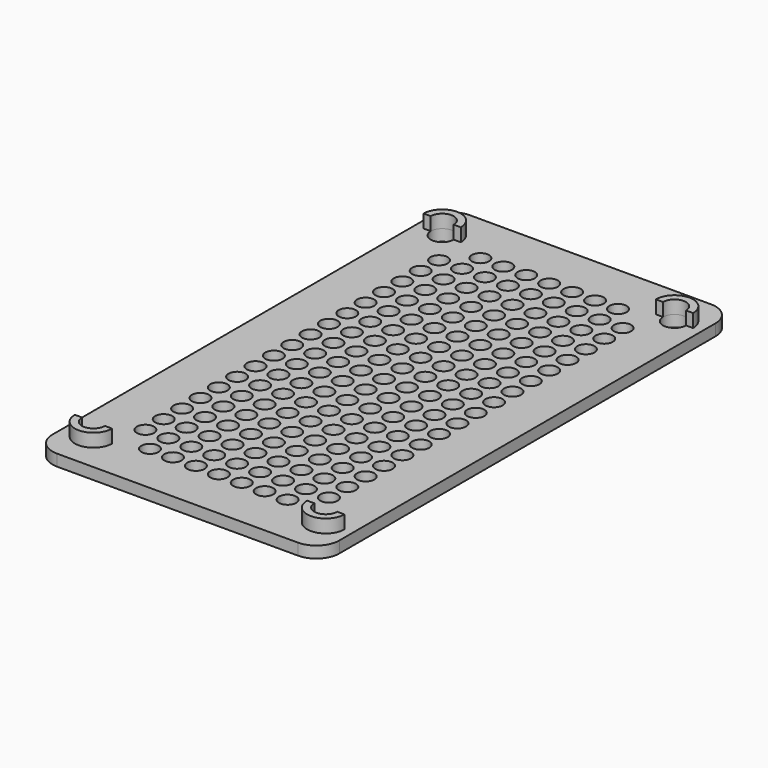
from build123d import *
from build123d import SkipClean  # not in build123d's __all__

# Parameters (mm, degrees)
F0_R     = 2
F0_R_2   = 1.5
F1_DEPTH = 2
F3_DEPTH = 2.3


with BuildPart() as f1:
    # F0 (on Top) → F1 (new body)
    with BuildSketch(Plane.XY):
        with BuildLine():
            Line((-21, -45), (21, -45))
            ThreePointArc((21, -45), (23.8284271247, -43.8284271247), (25, -41))
            Line((25, -41), (25, 41))
            ThreePointArc((25, 41), (23.8284271247, 43.8284271247), (21, 45))
            Line((21, 45), (-21, 45))
            ThreePointArc((-21, 45), (-23.8284271247, 43.8284271247), (-25, 41))
            Line((-25, 41), (-25, -41))
            ThreePointArc((-25, -41), (-23.8284271247, -43.8284271247), (-21, -45))
        make_face()
        with Locations((-20.25, -38)):
            Circle(F0_R, mode=Mode.SUBTRACT)
        with Locations((-16, -32)):
            Circle(F0_R_2, mode=Mode.SUBTRACT)
        with Locations((-16, -28)):
            Circle(F0_R_2, mode=Mode.SUBTRACT)
        with Locations((-16, -24)):
            Circle(F0_R_2, mode=Mode.SUBTRACT)
        with Locations((-12, -36)):
            Circle(F0_R_2, mode=Mode.SUBTRACT)
        with Locations((-8, -36)):
            Circle(F0_R_2, mode=Mode.SUBTRACT)
        with Locations((-4, -36)):
            Circle(F0_R_2, mode=Mode.SUBTRACT)
        with Locations((-12, -32)):
            Circle(F0_R_2, mode=Mode.SUBTRACT)
        with Locations((-8, -32)):
            Circle(F0_R_2, mode=Mode.SUBTRACT)
        with Locations((-12, -28)):
            Circle(F0_R_2, mode=Mode.SUBTRACT)
        with Locations((-12, -24)):
            Circle(F0_R_2, mode=Mode.SUBTRACT)
        with Locations((-8, -28)):
            Circle(F0_R_2, mode=Mode.SUBTRACT)
        with Locations((-8, -24)):
            Circle(F0_R_2, mode=Mode.SUBTRACT)
        with Locations((-4, -32)):
            Circle(F0_R_2, mode=Mode.SUBTRACT)
        with Locations((-4, -28)):
            Circle(F0_R_2, mode=Mode.SUBTRACT)
        with Locations((-4, -24)):
            Circle(F0_R_2, mode=Mode.SUBTRACT)
        with Locations((-16, -20)):
            Circle(F0_R_2, mode=Mode.SUBTRACT)
        with Locations((-16, -16)):
            Circle(F0_R_2, mode=Mode.SUBTRACT)
        with Locations((-16, -12)):
            Circle(F0_R_2, mode=Mode.SUBTRACT)
        with Locations((-16, -8)):
            Circle(F0_R_2, mode=Mode.SUBTRACT)
        with Locations((-16, -4)):
            Circle(F0_R_2, mode=Mode.SUBTRACT)
        with Locations((-12, -20)):
            Circle(F0_R_2, mode=Mode.SUBTRACT)
        with Locations((-8, -20)):
            Circle(F0_R_2, mode=Mode.SUBTRACT)
        with Locations((-12, -16)):
            Circle(F0_R_2, mode=Mode.SUBTRACT)
        with Locations((-12, -12)):
            Circle(F0_R_2, mode=Mode.SUBTRACT)
        with Locations((-8, -16)):
            Circle(F0_R_2, mode=Mode.SUBTRACT)
        with Locations((-8, -12)):
            Circle(F0_R_2, mode=Mode.SUBTRACT)
        with Locations((-4, -20)):
            Circle(F0_R_2, mode=Mode.SUBTRACT)
        with Locations((-4, -16)):
            Circle(F0_R_2, mode=Mode.SUBTRACT)
        with Locations((-4, -12)):
            Circle(F0_R_2, mode=Mode.SUBTRACT)
        with Locations((-12, -8)):
            Circle(F0_R_2, mode=Mode.SUBTRACT)
        with Locations((-8, -8)):
            Circle(F0_R_2, mode=Mode.SUBTRACT)
        with Locations((-12, -4)):
            Circle(F0_R_2, mode=Mode.SUBTRACT)
        with Locations((-8, -4)):
            Circle(F0_R_2, mode=Mode.SUBTRACT)
        with Locations((-4, -8)):
            Circle(F0_R_2, mode=Mode.SUBTRACT)
        with Locations((-4, -4)):
            Circle(F0_R_2, mode=Mode.SUBTRACT)
        with Locations((0, -36)):
            Circle(F0_R_2, mode=Mode.SUBTRACT)
        with Locations((4, -36)):
            Circle(F0_R_2, mode=Mode.SUBTRACT)
        with Locations((8, -36)):
            Circle(F0_R_2, mode=Mode.SUBTRACT)
        with Locations((12, -36)):
            Circle(F0_R_2, mode=Mode.SUBTRACT)
        with Locations((0, -32)):
            Circle(F0_R_2, mode=Mode.SUBTRACT)
        with Locations((4, -32)):
            Circle(F0_R_2, mode=Mode.SUBTRACT)
        with Locations((0, -28)):
            Circle(F0_R_2, mode=Mode.SUBTRACT)
        with Locations((0, -24)):
            Circle(F0_R_2, mode=Mode.SUBTRACT)
        with Locations((4, -28)):
            Circle(F0_R_2, mode=Mode.SUBTRACT)
        with Locations((4, -24)):
            Circle(F0_R_2, mode=Mode.SUBTRACT)
        with Locations((8, -32)):
            Circle(F0_R_2, mode=Mode.SUBTRACT)
        with Locations((12, -32)):
            Circle(F0_R_2, mode=Mode.SUBTRACT)
        with Locations((8, -28)):
            Circle(F0_R_2, mode=Mode.SUBTRACT)
        with Locations((8, -24)):
            Circle(F0_R_2, mode=Mode.SUBTRACT)
        with Locations((12, -28)):
            Circle(F0_R_2, mode=Mode.SUBTRACT)
        with Locations((12, -24)):
            Circle(F0_R_2, mode=Mode.SUBTRACT)
        with Locations((20.25, -38)):
            Circle(F0_R, mode=Mode.SUBTRACT)
        with Locations((16, -32)):
            Circle(F0_R_2, mode=Mode.SUBTRACT)
        with Locations((16, -28)):
            Circle(F0_R_2, mode=Mode.SUBTRACT)
        with Locations((16, -24)):
            Circle(F0_R_2, mode=Mode.SUBTRACT)
        with Locations((0, -20)):
            Circle(F0_R_2, mode=Mode.SUBTRACT)
        with Locations((4, -20)):
            Circle(F0_R_2, mode=Mode.SUBTRACT)
        with Locations((0, -16)):
            Circle(F0_R_2, mode=Mode.SUBTRACT)
        with Locations((0, -12)):
            Circle(F0_R_2, mode=Mode.SUBTRACT)
        with Locations((4, -16)):
            Circle(F0_R_2, mode=Mode.SUBTRACT)
        with Locations((4, -12)):
            Circle(F0_R_2, mode=Mode.SUBTRACT)
        with Locations((8, -20)):
            Circle(F0_R_2, mode=Mode.SUBTRACT)
        with Locations((12, -20)):
            Circle(F0_R_2, mode=Mode.SUBTRACT)
        with Locations((8, -16)):
            Circle(F0_R_2, mode=Mode.SUBTRACT)
        with Locations((8, -12)):
            Circle(F0_R_2, mode=Mode.SUBTRACT)
        with Locations((12, -16)):
            Circle(F0_R_2, mode=Mode.SUBTRACT)
        with Locations((12, -12)):
            Circle(F0_R_2, mode=Mode.SUBTRACT)
        with Locations((0, -8)):
            Circle(F0_R_2, mode=Mode.SUBTRACT)
        with Locations((4, -8)):
            Circle(F0_R_2, mode=Mode.SUBTRACT)
        with Locations((0, -4)):
            Circle(F0_R_2, mode=Mode.SUBTRACT)
        with Locations((4, -4)):
            Circle(F0_R_2, mode=Mode.SUBTRACT)
        with Locations((8, -8)):
            Circle(F0_R_2, mode=Mode.SUBTRACT)
        with Locations((12, -8)):
            Circle(F0_R_2, mode=Mode.SUBTRACT)
        with Locations((8, -4)):
            Circle(F0_R_2, mode=Mode.SUBTRACT)
        with Locations((12, -4)):
            Circle(F0_R_2, mode=Mode.SUBTRACT)
        with Locations((16, -20)):
            Circle(F0_R_2, mode=Mode.SUBTRACT)
        with Locations((16, -16)):
            Circle(F0_R_2, mode=Mode.SUBTRACT)
        with Locations((16, -12)):
            Circle(F0_R_2, mode=Mode.SUBTRACT)
        with Locations((16, -8)):
            Circle(F0_R_2, mode=Mode.SUBTRACT)
        with Locations((16, -4)):
            Circle(F0_R_2, mode=Mode.SUBTRACT)
        with Locations((-16, 0)):
            Circle(F0_R_2, mode=Mode.SUBTRACT)
        with Locations((-16, 4)):
            Circle(F0_R_2, mode=Mode.SUBTRACT)
        with Locations((-16, 8)):
            Circle(F0_R_2, mode=Mode.SUBTRACT)
        with Locations((-16, 12)):
            Circle(F0_R_2, mode=Mode.SUBTRACT)
        with Locations((-16, 16)):
            Circle(F0_R_2, mode=Mode.SUBTRACT)
        with Locations((-16, 20)):
            Circle(F0_R_2, mode=Mode.SUBTRACT)
        with Locations((-12, 0)):
            Circle(F0_R_2, mode=Mode.SUBTRACT)
        with Locations((-12, 4)):
            Circle(F0_R_2, mode=Mode.SUBTRACT)
        with Locations((-8, 0)):
            Circle(F0_R_2, mode=Mode.SUBTRACT)
        with Locations((-8, 4)):
            Circle(F0_R_2, mode=Mode.SUBTRACT)
        with Locations((-12, 8)):
            Circle(F0_R_2, mode=Mode.SUBTRACT)
        with Locations((-8, 8)):
            Circle(F0_R_2, mode=Mode.SUBTRACT)
        with Locations((-4, 0)):
            Circle(F0_R_2, mode=Mode.SUBTRACT)
        with Locations((-4, 4)):
            Circle(F0_R_2, mode=Mode.SUBTRACT)
        with Locations((-4, 8)):
            Circle(F0_R_2, mode=Mode.SUBTRACT)
        with Locations((-12, 12)):
            Circle(F0_R_2, mode=Mode.SUBTRACT)
        with Locations((-12, 16)):
            Circle(F0_R_2, mode=Mode.SUBTRACT)
        with Locations((-8, 12)):
            Circle(F0_R_2, mode=Mode.SUBTRACT)
        with Locations((-8, 16)):
            Circle(F0_R_2, mode=Mode.SUBTRACT)
        with Locations((-12, 20)):
            Circle(F0_R_2, mode=Mode.SUBTRACT)
        with Locations((-8, 20)):
            Circle(F0_R_2, mode=Mode.SUBTRACT)
        with Locations((-4, 12)):
            Circle(F0_R_2, mode=Mode.SUBTRACT)
        with Locations((-4, 16)):
            Circle(F0_R_2, mode=Mode.SUBTRACT)
        with Locations((-4, 20)):
            Circle(F0_R_2, mode=Mode.SUBTRACT)
        with Locations((-16, 24)):
            Circle(F0_R_2, mode=Mode.SUBTRACT)
        with Locations((-16, 28)):
            Circle(F0_R_2, mode=Mode.SUBTRACT)
        with Locations((-16, 32)):
            Circle(F0_R_2, mode=Mode.SUBTRACT)
        with Locations((-20.25, 38)):
            Circle(F0_R, mode=Mode.SUBTRACT)
        with Locations((-12, 24)):
            Circle(F0_R_2, mode=Mode.SUBTRACT)
        with Locations((-12, 28)):
            Circle(F0_R_2, mode=Mode.SUBTRACT)
        with Locations((-8, 24)):
            Circle(F0_R_2, mode=Mode.SUBTRACT)
        with Locations((-8, 28)):
            Circle(F0_R_2, mode=Mode.SUBTRACT)
        with Locations((-12, 32)):
            Circle(F0_R_2, mode=Mode.SUBTRACT)
        with Locations((-8, 32)):
            Circle(F0_R_2, mode=Mode.SUBTRACT)
        with Locations((-4, 24)):
            Circle(F0_R_2, mode=Mode.SUBTRACT)
        with Locations((-4, 28)):
            Circle(F0_R_2, mode=Mode.SUBTRACT)
        with Locations((-4, 32)):
            Circle(F0_R_2, mode=Mode.SUBTRACT)
        with Locations((-12, 36)):
            Circle(F0_R_2, mode=Mode.SUBTRACT)
        with Locations((-8, 36)):
            Circle(F0_R_2, mode=Mode.SUBTRACT)
        with Locations((-4, 36)):
            Circle(F0_R_2, mode=Mode.SUBTRACT)
        Circle(F0_R_2, mode=Mode.SUBTRACT)
        with Locations((0, 4)):
            Circle(F0_R_2, mode=Mode.SUBTRACT)
        with Locations((4, 0)):
            Circle(F0_R_2, mode=Mode.SUBTRACT)
        with Locations((4, 4)):
            Circle(F0_R_2, mode=Mode.SUBTRACT)
        with Locations((0, 8)):
            Circle(F0_R_2, mode=Mode.SUBTRACT)
        with Locations((4, 8)):
            Circle(F0_R_2, mode=Mode.SUBTRACT)
        with Locations((8, 0)):
            Circle(F0_R_2, mode=Mode.SUBTRACT)
        with Locations((8, 4)):
            Circle(F0_R_2, mode=Mode.SUBTRACT)
        with Locations((12, 0)):
            Circle(F0_R_2, mode=Mode.SUBTRACT)
        with Locations((12, 4)):
            Circle(F0_R_2, mode=Mode.SUBTRACT)
        with Locations((8, 8)):
            Circle(F0_R_2, mode=Mode.SUBTRACT)
        with Locations((12, 8)):
            Circle(F0_R_2, mode=Mode.SUBTRACT)
        with Locations((0, 12)):
            Circle(F0_R_2, mode=Mode.SUBTRACT)
        with Locations((0, 16)):
            Circle(F0_R_2, mode=Mode.SUBTRACT)
        with Locations((4, 12)):
            Circle(F0_R_2, mode=Mode.SUBTRACT)
        with Locations((4, 16)):
            Circle(F0_R_2, mode=Mode.SUBTRACT)
        with Locations((0, 20)):
            Circle(F0_R_2, mode=Mode.SUBTRACT)
        with Locations((4, 20)):
            Circle(F0_R_2, mode=Mode.SUBTRACT)
        with Locations((8, 12)):
            Circle(F0_R_2, mode=Mode.SUBTRACT)
        with Locations((8, 16)):
            Circle(F0_R_2, mode=Mode.SUBTRACT)
        with Locations((12, 12)):
            Circle(F0_R_2, mode=Mode.SUBTRACT)
        with Locations((12, 16)):
            Circle(F0_R_2, mode=Mode.SUBTRACT)
        with Locations((8, 20)):
            Circle(F0_R_2, mode=Mode.SUBTRACT)
        with Locations((12, 20)):
            Circle(F0_R_2, mode=Mode.SUBTRACT)
        with Locations((16, 0)):
            Circle(F0_R_2, mode=Mode.SUBTRACT)
        with Locations((16, 4)):
            Circle(F0_R_2, mode=Mode.SUBTRACT)
        with Locations((16, 8)):
            Circle(F0_R_2, mode=Mode.SUBTRACT)
        with Locations((16, 12)):
            Circle(F0_R_2, mode=Mode.SUBTRACT)
        with Locations((16, 16)):
            Circle(F0_R_2, mode=Mode.SUBTRACT)
        with Locations((16, 20)):
            Circle(F0_R_2, mode=Mode.SUBTRACT)
        with Locations((0, 24)):
            Circle(F0_R_2, mode=Mode.SUBTRACT)
        with Locations((0, 28)):
            Circle(F0_R_2, mode=Mode.SUBTRACT)
        with Locations((4, 24)):
            Circle(F0_R_2, mode=Mode.SUBTRACT)
        with Locations((4, 28)):
            Circle(F0_R_2, mode=Mode.SUBTRACT)
        with Locations((0, 32)):
            Circle(F0_R_2, mode=Mode.SUBTRACT)
        with Locations((4, 32)):
            Circle(F0_R_2, mode=Mode.SUBTRACT)
        with Locations((8, 24)):
            Circle(F0_R_2, mode=Mode.SUBTRACT)
        with Locations((8, 28)):
            Circle(F0_R_2, mode=Mode.SUBTRACT)
        with Locations((12, 24)):
            Circle(F0_R_2, mode=Mode.SUBTRACT)
        with Locations((12, 28)):
            Circle(F0_R_2, mode=Mode.SUBTRACT)
        with Locations((8, 32)):
            Circle(F0_R_2, mode=Mode.SUBTRACT)
        with Locations((12, 32)):
            Circle(F0_R_2, mode=Mode.SUBTRACT)
        with Locations((0, 36)):
            Circle(F0_R_2, mode=Mode.SUBTRACT)
        with Locations((4, 36)):
            Circle(F0_R_2, mode=Mode.SUBTRACT)
        with Locations((8, 36)):
            Circle(F0_R_2, mode=Mode.SUBTRACT)
        with Locations((12, 36)):
            Circle(F0_R_2, mode=Mode.SUBTRACT)
        with Locations((16, 24)):
            Circle(F0_R_2, mode=Mode.SUBTRACT)
        with Locations((16, 28)):
            Circle(F0_R_2, mode=Mode.SUBTRACT)
        with Locations((16, 32)):
            Circle(F0_R_2, mode=Mode.SUBTRACT)
        with Locations((20.25, 38)):
            Circle(F0_R, mode=Mode.SUBTRACT)
    extrude(amount=F1_DEPTH)

    # F2 (on face) → F3 (join)
    with BuildSketch(Plane.XY.offset(2)):
        with BuildLine():
            ThreePointArc((-22.25, 38), (-20.25, 40), (-18.25, 38))
            Line((-18.25, 38), (-17.0000013254, 38))
            ThreePointArc((-17.0000013254, 38), (-20.25, 41.2499986746), (-23.4999986746, 38))
            Line((-23.4999986746, 38), (-22.25, 38))
        make_face()
        with BuildLine():
            ThreePointArc((23.4999986746, 38), (20.25, 41.2499986746), (17.0000013254, 38))
            Line((17.0000013254, 38), (18.25, 38))
            ThreePointArc((18.25, 38), (20.25, 40), (22.25, 38))
            Line((22.25, 38), (23.4999986746, 38))
        make_face()
        with BuildLine():
            Line((18.25, -38), (17.0000013254, -38))
            ThreePointArc((17.0000013254, -38), (20.25, -41.2499986746), (23.4999986746, -38))
            Line((23.4999986746, -38), (22.25, -38))
            ThreePointArc((22.25, -38), (20.25, -40), (18.25, -38))
        make_face()
        with BuildLine():
            ThreePointArc((-23.4999986746, -38), (-20.25, -41.2499986746), (-17.0000013254, -38))
            Line((-17.0000013254, -38), (-18.25, -38))
            ThreePointArc((-18.25, -38), (-20.25, -40), (-22.25, -38))
            Line((-22.25, -38), (-23.4999986746, -38))
        make_face()
    with SkipClean():  # cleaning this boolean's faces spoils the solid; the shape is the same uncleaned
        extrude(amount=F3_DEPTH)


solid = f1.part
